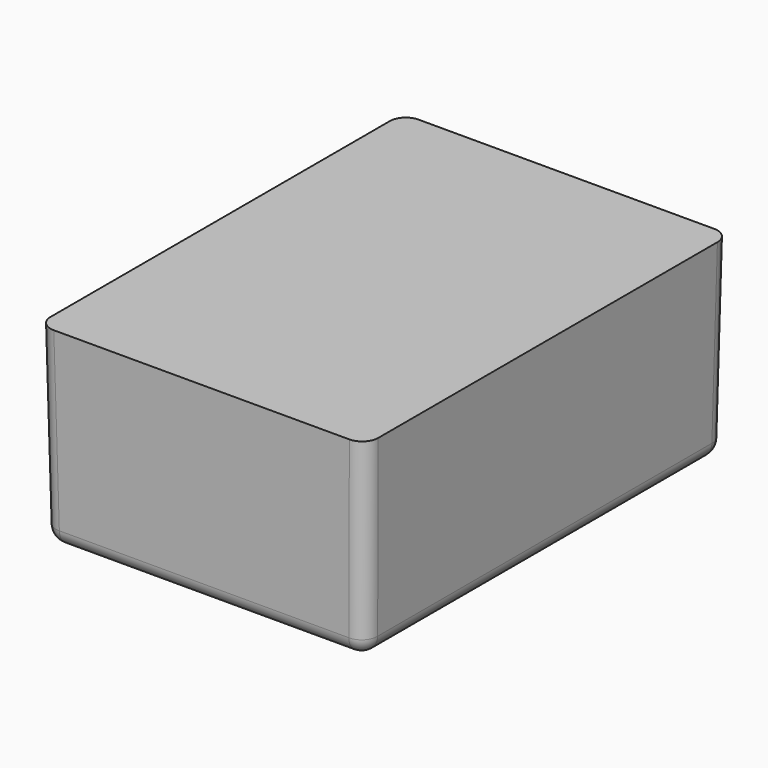
from build123d import *

# Parameters (mm, degrees)
F0_W     = 127
F0_H     = 177.8
F1_DEPTH = 76.2
F1_TAPER = -1
F3_R     = 6.35


# Not quite as in the source:
# - a feature of the source that left no trace in its solid (it failed there, or was rolled back) is left out


with BuildPart() as f1:
    # F0 (on Top) → F1 (new body)
    with BuildSketch(Plane.XY):
        Rectangle(F0_W, F0_H)
    extrude(amount=F1_DEPTH, taper=F1_TAPER)

    # F3
    f3_edges = [f1.edges().sort_by_distance(p)[0] for p in [
        (63.5, 0, 0),
        (0, -88.9, 0),
        (64.165038, -89.565038, 38.1),
        (-64.165038, -89.565038, 38.1),
        (64.165038, 89.565038, 38.1),
        (0, 88.9, 0),
        (-64.165038, 89.565038, 38.1),
        (-63.5, 0, 0),
    ]]
    fillet(f3_edges, radius=F3_R)


solid = f1.part
